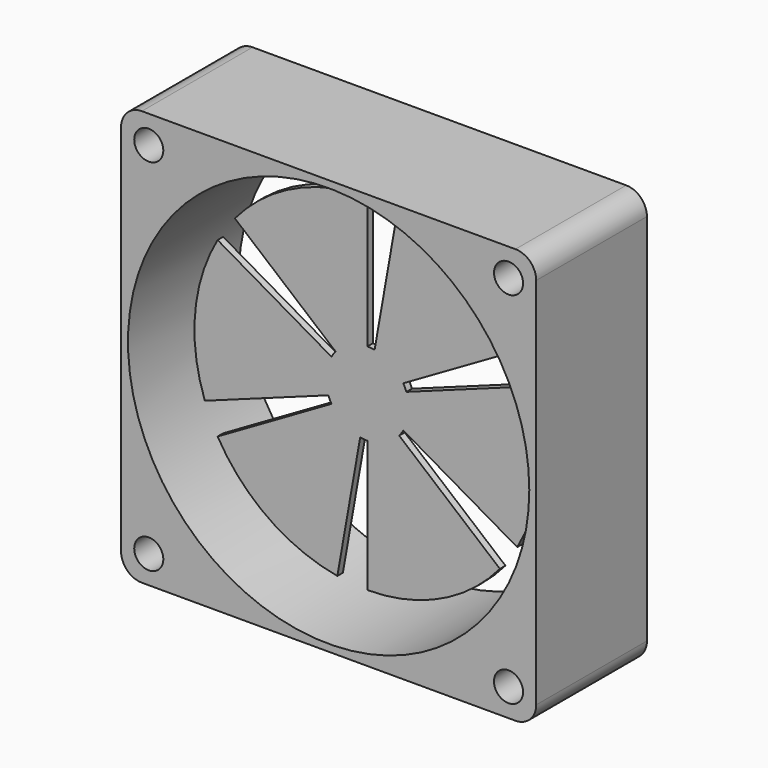
from build123d import *

# Parameters (mm, degrees)
F1_START = -7
F1_DEPTH = 1
F0_R     = 29
F2_DEPTH = 20
F3_D     = 4.2


# Not quite as in the source:
# - a feature names something its author has since deleted; it is built from what else it names


with BuildPart() as f1:
    # F0 (on Front) → F1 (new body)
    with BuildSketch(Plane.XZ.offset(F1_START)):
        with BuildLine():
            Line((4.3412044417, 24.6201938253), (1.041889066, 5.9088465181))
            ThreePointArc((1.041889066, 5.9088465181), (3.4414586181, 4.9149122657), (5.1961524227, 3))
            Line((5.1961524227, 3), (21.6506350946, 12.5))
            ThreePointArc((21.6506350946, 12.5), (14.3394109088, 20.4788011072), (4.3412044417, 24.6201938253))
        make_face()
        with BuildLine():
            ThreePointArc((1.041889066, 5.9088465181), (0.5229344565, 5.9771681886), (0, 6))
            ThreePointArc((0, 6), (-2.5357095704, 5.4378467222), (-4.5962666587, 3.8567256581))
            ThreePointArc((-4.5962666587, 3.8567256581), (-4.9149122657, 3.4414586181), (-5.1961524227, 3))
            ThreePointArc((-5.1961524227, 3), (-5.9771681886, 0.5229344565), (-5.6381557247, -2.05212086))
            ThreePointArc((-5.6381557247, -2.05212086), (-5.4378467222, -2.5357095704), (-5.1961524227, -3))
            ThreePointArc((-5.1961524227, -3), (-3.4414586181, -4.9149122657), (-1.041889066, -5.9088465181))
            ThreePointArc((-1.041889066, -5.9088465181), (-0.5229344565, -5.9771681886), (0, -6))
            ThreePointArc((0, -6), (2.5357095704, -5.4378467222), (4.5962666587, -3.8567256581))
            ThreePointArc((4.5962666587, -3.8567256581), (4.9149122657, -3.4414586181), (5.1961524227, -3))
            ThreePointArc((5.1961524227, -3), (5.7955549577, -1.5529142706), (6, 0))
            ThreePointArc((6, 0), (5.9088465181, 1.041889066), (5.6381557247, 2.05212086))
            ThreePointArc((5.6381557247, 2.05212086), (5.4378467222, 2.5357095704), (5.1961524227, 3))
            ThreePointArc((5.1961524227, 3), (3.4414586181, 4.9149122657), (1.041889066, 5.9088465181))
        make_face()
        with BuildLine():
            Line((0, 6), (0, 25))
            ThreePointArc((0, 25), (-10.5654564932, 22.6576945681), (-19.151111078, 16.0696902422))
            Line((-19.151111078, 16.0696902422), (-4.5962666587, 3.8567256581))
            ThreePointArc((-4.5962666587, 3.8567256581), (-2.5357095704, 5.4378467222), (0, 6))
        make_face()
        with BuildLine():
            ThreePointArc((-5.6381557247, -2.05212086), (-5.9771681886, 0.5229344565), (-5.1961524227, 3))
            Line((-5.1961524227, 3), (-21.6506350946, 12.5))
            ThreePointArc((-21.6506350946, 12.5), (-24.9048674523, 2.1788935687), (-23.4923155196, -8.5505035831))
            Line((-23.4923155196, -8.5505035831), (-5.6381557247, -2.05212086))
        make_face()
        with BuildLine():
            ThreePointArc((-1.041889066, -5.9088465181), (-3.4414586181, -4.9149122657), (-5.1961524227, -3))
            Line((-5.1961524227, -3), (-21.6506350946, -12.5))
            ThreePointArc((-21.6506350946, -12.5), (-14.3394109088, -20.4788011072), (-4.3412044417, -24.6201938253))
            Line((-4.3412044417, -24.6201938253), (-1.041889066, -5.9088465181))
        make_face()
        with BuildLine():
            ThreePointArc((4.5962666587, -3.8567256581), (2.5357095704, -5.4378467222), (0, -6))
            Line((0, -6), (0, -25))
            ThreePointArc((0, -25), (10.5654565435, -22.6576946759), (19.151111078, -16.0696902422))
            Line((19.151111078, -16.0696902422), (4.5962666587, -3.8567256581))
        make_face()
        with BuildLine():
            Line((23.4923155196, 8.5505035831), (5.6381557247, 2.05212086))
            ThreePointArc((5.6381557247, 2.05212086), (5.9088465181, 1.041889066), (6, 0))
            ThreePointArc((6, 0), (5.7955549577, -1.5529142706), (5.1961524227, -3))
            Line((5.1961524227, -3), (21.6506350946, -12.5))
            ThreePointArc((21.6506350946, -12.5), (24.9048674523, -2.1788935687), (23.4923155196, 8.5505035831))
        make_face()
    extrude(amount=-F1_DEPTH)


with BuildPart() as f2:
    # F0 (on Front) → F2 (new body)
    with BuildSketch(Plane.XZ):
        with BuildLine():
            Line((30, -27), (30, 27))
            ThreePointArc((30, 27), (29.1213203436, 29.1213203436), (27, 30))
            Line((27, 30), (-27, 30))
            ThreePointArc((-27, 30), (-29.1213203436, 29.1213203436), (-30, 27))
            Line((-30, 27), (-30, -27))
            ThreePointArc((-30, -27), (-29.1213203436, -29.1213203436), (-27, -30))
            Line((-27, -30), (27, -30))
            ThreePointArc((27, -30), (29.1213203436, -29.1213203436), (30, -27))
        make_face()
        Circle(F0_R, mode=Mode.SUBTRACT)
    extrude(amount=-F2_DEPTH)

    # F3 (through all)
    with Locations(Plane.XZ):
        with Locations((-26, 26), (26, 26), (26, -26), (-26, -26)):
            Hole(F3_D / 2)


solid = Compound([f1.part, f2.part])
